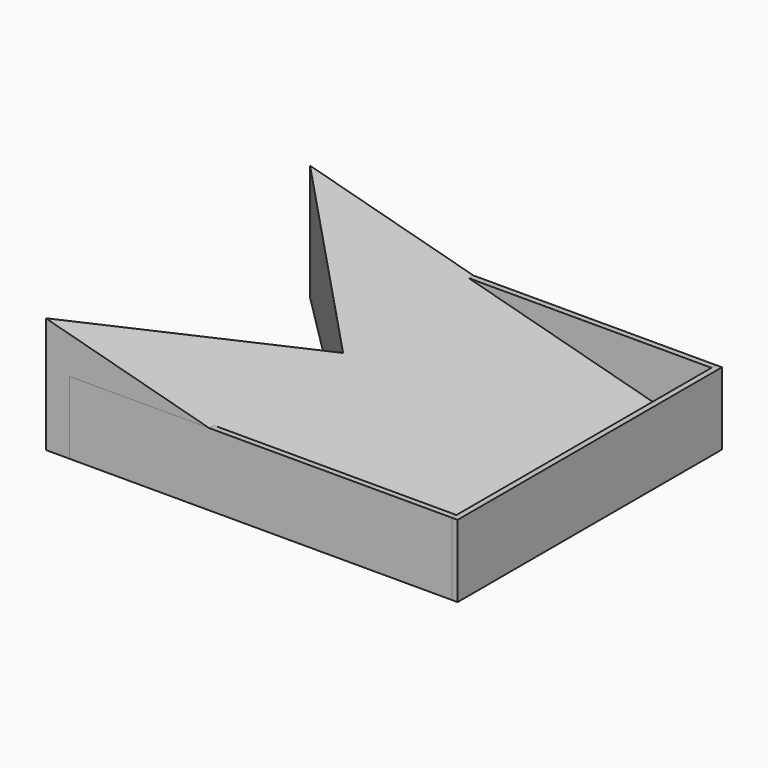
from build123d import *

# Parameters (mm, degrees)
F1_DEPTH  = 57
F2_W      = 57
F2_H      = 12.5
F3_DEPTH  = 1
F4_W      = 66
F4_H      = 12.5
F5_DEPTH  = 1
F7_W      = 66
F7_H      = 12.5
F8_DEPTH  = 1
F10_DEPTH = 25


# Not quite as in the source:
# - a feature names something its author has since deleted; it is built from what else it names


with BuildPart() as f1:
    # F0 (on Front) → F1 (new body)
    with BuildSketch(Plane.XZ):
        Polygon((-70, 0), (0, 0), (0, 1.33974), (-70, 20), align=None)
    extrude(amount=-F1_DEPTH)

    # F9 (on Top) → F10 (cut)
    with BuildSketch(Plane.XY):
        Polygon((-70.0584907394, 57), (-70.0584907394, 0), (-41.5584907394, 28.5), align=None)
    extrude(amount=F10_DEPTH, mode=Mode.SUBTRACT)


with BuildPart() as f3:
    # F2 (on Right) → F3 (new body)
    with BuildSketch(Plane.YZ):
        with Locations((28.5, 6.25)):
            Rectangle(F2_W, F2_H)
    extrude(amount=F3_DEPTH)


with BuildPart() as f5:
    # F4 (on Front) → F5 (new body)
    with BuildSketch(Plane.XZ):
        with Locations((-33, 6.25)):
            Rectangle(F4_W, F4_H)
    extrude(amount=-F5_DEPTH)


with BuildPart() as f8:
    # F7 (on offset) → F8 (new body)
    with BuildSketch(Plane(origin=(0, 57, 0), x_dir=(-1, 0, 0), z_dir=(0, 1, 0))):
        with Locations((33, 6.25)):
            Rectangle(F7_W, F7_H)
    extrude(amount=-F8_DEPTH)


solid = Compound([f1.part, f3.part, f5.part, f8.part])
